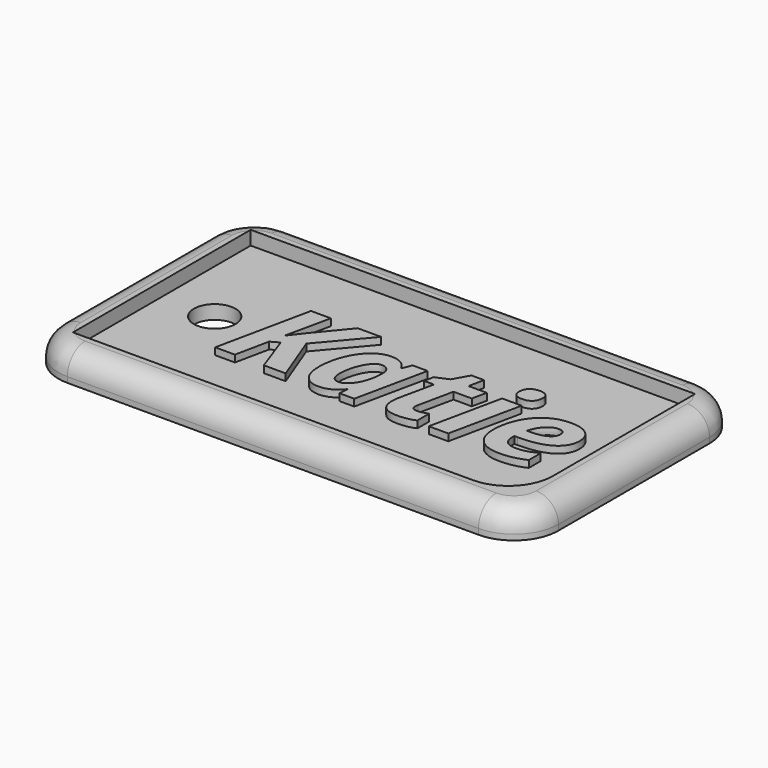
from build123d import *

# Parameters (mm, degrees)
F0_W         = 57.15
F0_H         = 31.75
F0_W_2       = 50.8
F0_H_2       = 25.4
F0_R         = 2.38125
F1_DEPTH     = 1.5875
F2_DEPTH     = 3.175
F3_R         = 5.08
F4_T1_DEPTH  = 46.99
F4_T3_DEPTH  = 21.59
F4_T6_ANGLE  = 90
F4_T8_ANGLE  = 90
F4_T10_ANGLE = 90
F4_T12_ANGLE = 90
F5_TEXT_SIZE = 15.1726712712
F6_DEPTH     = 0.79375


# Not quite as in the source:
# - a fillet or chamfer that OpenCascade refuses, or shapes differently, is made with other operations: its cross-section is extruded or revolved along the edge and cut away or added
# - Text() gives the source's letters only with a copy of the font that has no kerning and outlines rounded to 1/6400 em; it was checked with that copy


with BuildPart() as f1:
    # F0 (on Top) → F1 (new body)
    with BuildSketch(Plane.XY):
        with Locations((25.4, 12.7)):
            Rectangle(F0_W, F0_H)
        with Locations((25.4, 12.7)):
            Rectangle(F0_W_2, F0_H_2, mode=Mode.SUBTRACT)
        with Locations((25.4, 12.7)):
            Rectangle(F0_W_2, F0_H_2)
        with Locations((6.0472679324, 12.7)):
            Circle(F0_R, mode=Mode.SUBTRACT)
    extrude(amount=F1_DEPTH)

    # F0 (on Top) → F2 (join)
    with BuildSketch(Plane.XY):
        with Locations((25.4, 12.7)):
            Rectangle(F0_W, F0_H)
        with Locations((25.4, 12.7)):
            Rectangle(F0_W_2, F0_H_2, mode=Mode.SUBTRACT)
    extrude(amount=F2_DEPTH)

    # F3
    f3_edges = [f1.edges().sort_by_distance(p)[0] for p in [
        (53.975, -3.175, 1.5875),
        (-3.175, -3.175, 1.5875),
        (50.8, 0, 2.38125),
        (53.975, 28.575, 1.5875),
        (-3.175, 28.575, 1.5875),
    ]]
    fillet(f3_edges, radius=F3_R)

    # F4: fillet of radius 2.54 on 8 edges, made by hand

    # F4_s2 → F4_t1 (cut)
    with BuildSketch(Plane.YZ.offset(1.905)):
        with BuildLine():
            ThreePointArc((-0.635, 3.175), (-2.4310512242, 2.4310512242), (-3.175, 0.635))
            Line((-3.175, 0.635), (-3.175, 3.175))
            Line((-3.175, 3.175), (-0.635, 3.175))
        make_face()
        with BuildLine():
            ThreePointArc((28.575, 0.635), (27.8310512242, 2.4310512242), (26.035, 3.175))
            Line((26.035, 3.175), (28.575, 3.175))
            Line((28.575, 3.175), (28.575, 0.635))
        make_face()
    extrude(amount=F4_T1_DEPTH, mode=Mode.SUBTRACT)

    # F4_s4 → F4_t3 (cut)
    with BuildSketch(Plane.XZ.offset(-23.495)):
        with BuildLine():
            ThreePointArc((51.435, 3.175), (53.2310512242, 2.4310512242), (53.975, 0.635))
            Line((53.975, 0.635), (53.975, 3.175))
            Line((53.975, 3.175), (51.435, 3.175))
        make_face()
        with BuildLine():
            ThreePointArc((-0.635, 3.175), (-2.4310512242, 2.4310512242), (-3.175, 0.635))
            Line((-3.175, 0.635), (-3.175, 3.175))
            Line((-3.175, 3.175), (-0.635, 3.175))
        make_face()
    extrude(amount=F4_T3_DEPTH, mode=Mode.SUBTRACT)

    # F4_s5 → F4_t6 (revolve, cut)
    with BuildSketch(Plane.YZ.offset(48.895)):
        with BuildLine():
            ThreePointArc((26.035, 3.175), (27.8310512242, 2.4310512242), (28.575, 0.635))
            Line((28.575, 0.635), (28.575, 3.175))
            Line((28.575, 3.175), (26.035, 3.175))
        make_face()
    revolve(axis=Axis((48.895, 23.495, 3.175), (0, 0, -1)), revolution_arc=F4_T6_ANGLE, mode=Mode.SUBTRACT)

    # F4_s7 → F4_t8 (revolve, cut)
    with BuildSketch(Plane.YZ.offset(1.905)):
        with BuildLine():
            ThreePointArc((26.035, 3.175), (27.8310512242, 2.4310512242), (28.575, 0.635))
            Line((28.575, 0.635), (28.575, 3.175))
            Line((28.575, 3.175), (26.035, 3.175))
        make_face()
    revolve(axis=Axis((1.905, 23.495, 3.175), (0, 0, 1)), revolution_arc=F4_T8_ANGLE, mode=Mode.SUBTRACT)

    # F4_s9 → F4_t10 (revolve, cut)
    with BuildSketch(Plane.YZ.offset(48.895)):
        with BuildLine():
            ThreePointArc((-0.635, 3.175), (-2.4310512242, 2.4310512242), (-3.175, 0.635))
            Line((-3.175, 0.635), (-3.175, 3.175))
            Line((-3.175, 3.175), (-0.635, 3.175))
        make_face()
    revolve(axis=Axis((48.895, 1.905, 3.175), (0, 0, 1)), revolution_arc=F4_T10_ANGLE, mode=Mode.SUBTRACT)

    # F4_s11 → F4_t12 (revolve, cut)
    with BuildSketch(Plane.YZ.offset(1.905)):
        with BuildLine():
            ThreePointArc((-0.635, 3.175), (-2.4310512242, 2.4310512242), (-3.175, 0.635))
            Line((-3.175, 0.635), (-3.175, 3.175))
            Line((-3.175, 3.175), (-0.635, 3.175))
        make_face()
    revolve(axis=Axis((1.905, 1.905, 3.175), (0, 0, -1)), revolution_arc=F4_T12_ANGLE, mode=Mode.SUBTRACT)

    # F5 (on face) → F6 (join)
    with BuildSketch(Plane.XY.offset(1.5875)):
        with Locations((10.3721389427, 6.8685161957)):
            Text('Katie', F5_TEXT_SIZE, font='Open Sans', font_style=FontStyle.BOLDITALIC, text_align=(TextAlign.LEFT, TextAlign.BOTTOM))
    extrude(amount=F6_DEPTH)


solid = f1.part
